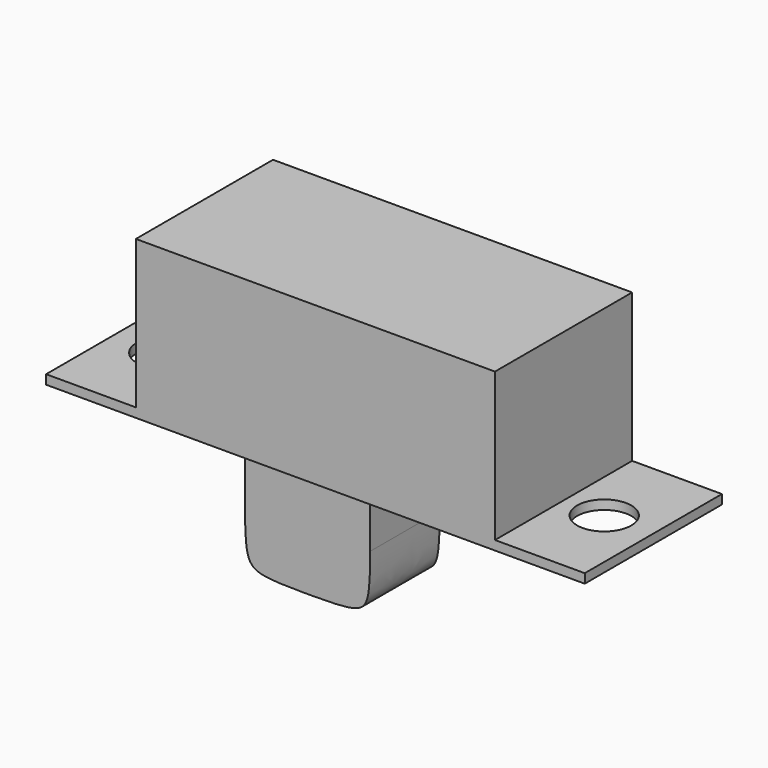
from build123d import *

# Parameters (mm, degrees)
F0_W        = 3.875
F0_H        = 7.4
F0_R        = 1.17
F0_W_2      = 15.5
F1_DEPTH    = 0.4
F2_DEPTH    = 6.4
F3_W        = 3.6
F3_H        = 3.75
F4_DEPTH    = 0.5
F3_W_2      = 5.4
F5_DEPTH    = 5.5
F6_T1_DEPTH = 16.25
F7_DEPTH    = 0.5


# Not quite as in the source:
# - a fillet or chamfer that OpenCascade refuses, or shapes differently, is made with other operations: its cross-section is extruded or revolved along the edge and cut away or added


with BuildPart() as f1:
    # F0 (on Top) → F1 (new body)
    with BuildSketch(Plane.XY):
        with Locations((-9.6875, 0)):
            Rectangle(F0_W, F0_H)
        with Locations((-9.505, 0)):
            Circle(F0_R, mode=Mode.SUBTRACT)
        Rectangle(F0_W_2, F0_H)
        with Locations((9.6875, 0)):
            Rectangle(F0_W, F0_H)
        with Locations((9.505, 0)):
            Circle(F0_R, mode=Mode.SUBTRACT)
    extrude(amount=-F1_DEPTH)

    # F0 (on Top) → F2 (join)
    with BuildSketch(Plane.XY):
        Rectangle(F0_W_2, F0_H)
    extrude(amount=F2_DEPTH)

    # F3 (on face) → F4 (cut)
    with BuildSketch(Plane(origin=(0, 0, -0.4), x_dir=(1, 0, 0), z_dir=(0, 0, -1))):
        with Locations((2.7, 0)):
            Rectangle(F3_W, F3_H)
    extrude(amount=-F4_DEPTH, mode=Mode.SUBTRACT)

    # F3 (on face) → F5 (join)
    with BuildSketch(Plane(origin=(0, 0, -0.4), x_dir=(1, 0, 0), z_dir=(0, 0, -1))):
        with Locations((-1.8, 0)):
            Rectangle(F3_W_2, F3_H)
    extrude(amount=F5_DEPTH)

    # F6: fillet of radius 2.5 on 2 edges, made by hand

    # F6_s2 → F6_t1 (cut)
    with BuildSketch(Plane.XZ.offset(-8.125)):
        with BuildLine():
            add(Edge.make_bspline(
                [(-4.5, -3.4), (-4.5, -5.9), (-2, -5.9)],
                knots=[0, 0, 0, 1, 1, 1], degree=2, weights=[1, 3, 1]))
            Line((-2, -5.9), (-4.5, -5.9))
            Line((-4.5, -5.9), (-4.5, -3.4))
        make_face()
        with BuildLine():
            add(Edge.make_bspline(
                [(0.9, -3.4), (0.9, -5.9), (-1.6, -5.9)],
                knots=[0, 0, 0, 1, 1, 1], degree=2, weights=[1, 3, 1]))
            Line((-1.6, -5.9), (0.9, -5.9))
            Line((0.9, -5.9), (0.9, -3.4))
        make_face()
    extrude(amount=F6_T1_DEPTH, mode=Mode.SUBTRACT)

    # F3 (on face) → F7 (cut)
    with BuildSketch(Plane(origin=(0, 0, -0.4), x_dir=(1, 0, 0), z_dir=(0, 0, -1))):
        with Locations((2.7, 0)):
            Rectangle(F3_W, F3_H)
    extrude(amount=-F7_DEPTH, mode=Mode.SUBTRACT)


solid = f1.part
